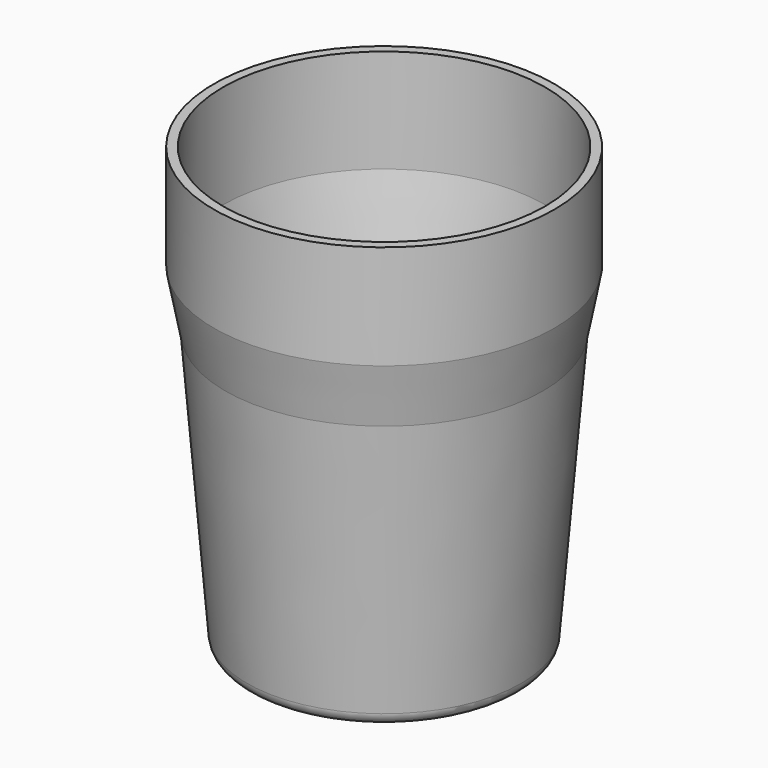
from build123d import *

# Parameters (mm, degrees)
F2_SIZE = 0.99999
F3_R    = 3
F4_R    = 1
F5_R    = 0.99999


# Not quite as in the source:
# - a fillet or chamfer is up to 0.001 mm smaller than in the source, because OpenCascade refuses the exact size


with BuildPart() as f1:
    # F0 (on Front) → F1 (revolve)
    with BuildSketch(Plane.XZ):
        Polygon((0, 2), (0, 0), (10.6, 0), (10.6, -1), (30, -1), (35, 60), (37.5, 73), (37.5, 96), (35.5, 96), (35.5, 73.1905618359), (33.0155331198, 60.2713340591), (28.1572270494, 1), (12.6, 1), (12.6, 2), align=None)
    revolve(axis=Axis((0, 0, 49), (0, 0, 1)))

    # F2 (size 1 in the source; OpenCascade refuses exactly that, so slightly less here)
    f2_edges = [f1.edges().sort_by_distance(p)[0] for p in [
        (-10.6, 0, -1),
    ]]
    chamfer(f2_edges, length=F2_SIZE)

    # F3
    f3_edges = [f1.edges().sort_by_distance(p)[0] for p in [
        (-30, 0, -1),
    ]]
    fillet(f3_edges, radius=F3_R)

    # F4
    f4_edges = [f1.edges().sort_by_distance(p)[0] for p in [
        (-28.157227, 0, 1),
    ]]
    fillet(f4_edges, radius=F4_R)

    # F5 (radius 1 in the source; OpenCascade refuses exactly that, so slightly less here)
    f5_edges = [f1.edges().sort_by_distance(p)[0] for p in [
        (-12.6, 0, 1),
    ]]
    fillet(f5_edges, radius=F5_R)


solid = f1.part
